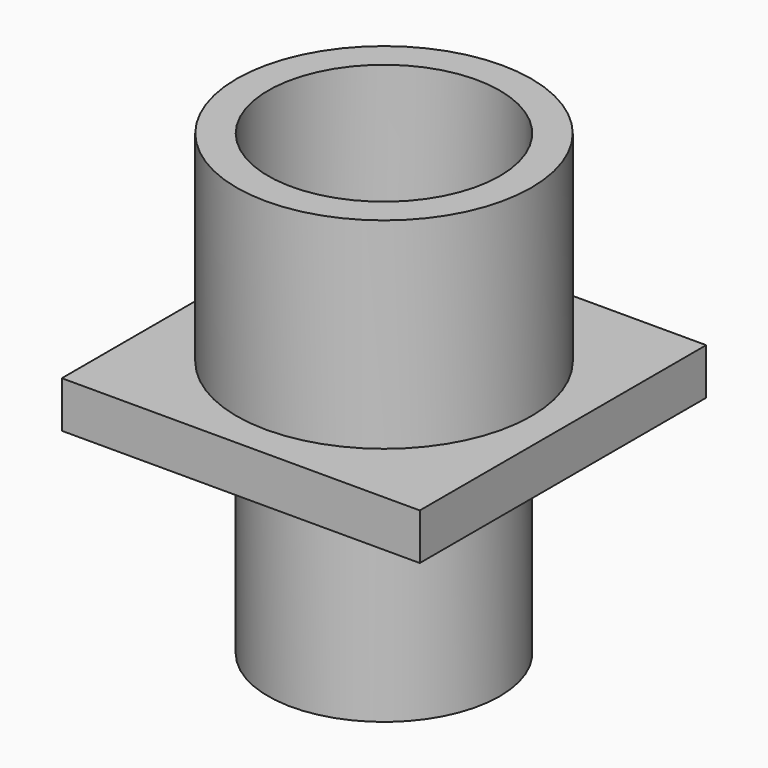
from build123d import *

# Parameters (mm, degrees)
F0_W     = 170
F0_H     = 170
F1_DEPTH = 17.5
F2_R     = 70
F2_R_2   = 55
F3_DEPTH = 100
F4_W     = 170
F4_H     = 170
F5_DEPTH = 22
F6_R     = 55
F7_DEPTH = 100


with BuildPart() as f1:
    # F0 (on Top) → F1 (new body)
    with BuildSketch(Plane.XY):
        Rectangle(F0_W, F0_H)
    extrude(amount=F1_DEPTH)

    # F2 (on face) → F3 (join)
    with BuildSketch(Plane.XY.offset(17.5)):
        Circle(F2_R)
        Circle(F2_R_2, mode=Mode.SUBTRACT)
    extrude(amount=F3_DEPTH)


with BuildPart() as f5:
    # F4 (on Top) → F5 (new body)
    with BuildSketch(Plane.XY):
        Rectangle(F4_W, F4_H)
    extrude(amount=F5_DEPTH)

    # F6 (on face) → F7 (join)
    with BuildSketch(Plane(origin=(0, 0, 0), x_dir=(1, 0, 0), z_dir=(0, 0, -1))):
        Circle(F6_R)
    extrude(amount=F7_DEPTH)


solid = Compound([f1.part, f5.part])
